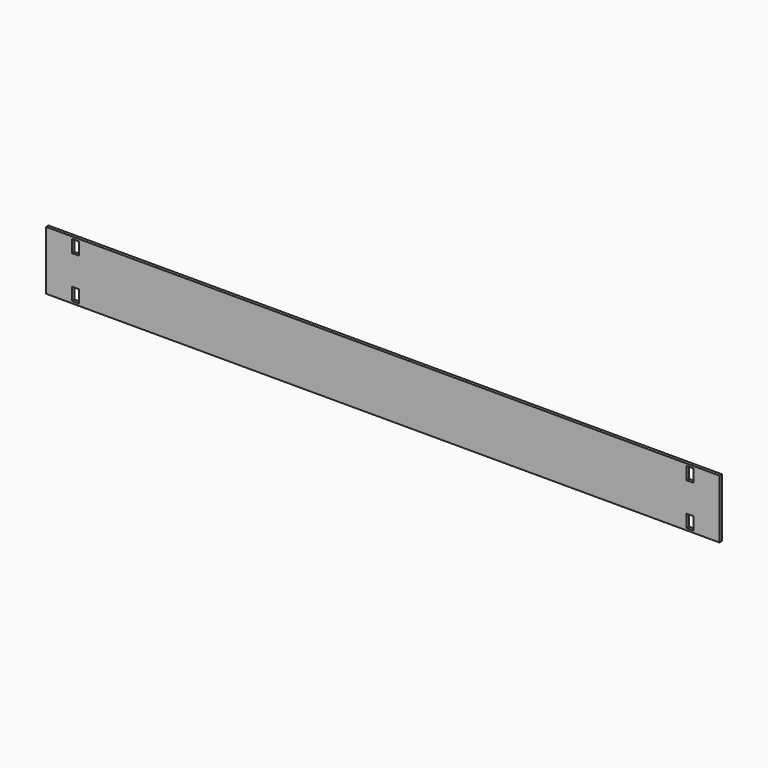
from build123d import *

# Parameters (mm, degrees)
F0_W     = 508
F0_H     = 44.45
F1_DEPTH = 2.286
F2_W     = 5.08
F2_H     = 9.525
F3_DEPTH = 2.287


# Not quite as in the source:
# - a pattern or mirror of a feature is missing from the dataset's text; its kind, count and spacing are read off the source's solid


with BuildPart() as f1:
    # F0 (on Front) → F1 (new body)
    with BuildSketch(Plane.XZ):
        Rectangle(F0_W, F0_H)
    extrude(amount=F1_DEPTH)

    # F2 (on face) → F3 (cut, through all)
    with BuildSketch(Plane.XZ.offset(2.286)):
        with Locations((-231.775, 15.875)):
            Rectangle(F2_W, F2_H)
        with Locations((-231.775, -15.875)):
            Rectangle(F2_W, F2_H)
    f3 = extrude(amount=-F3_DEPTH, mode=Mode.SUBTRACT)

    # F3_copies: F3 across plane
    add(f3.mirror(Plane(origin=(0, 0, 0), x_dir=(0, 0, 1), z_dir=(1, 0, 0))), mode=Mode.SUBTRACT)


solid = f1.part
